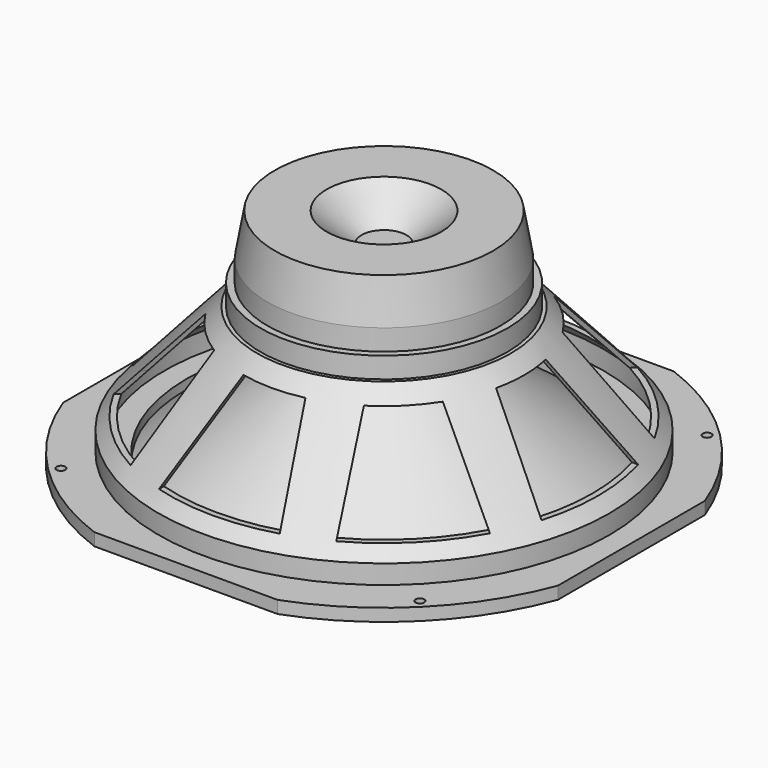
from build123d import *

# Parameters (mm, degrees)
F0_W            = 309.62
F0_H            = 309.62
F3_DEPTH        = 140.601
F5_D            = 5.5
F5_COPIES_COUNT = 4
F6_DEPTH        = 154.811
F6_COPIES_COUNT = 8


# Not quite as in the source:
# - a pattern or mirror of a feature is missing from the dataset's text; its kind, count and spacing are read off the source's solid


with BuildPart() as f2:
    # F1 (on Front) → F2 (revolve)
    with BuildSketch(Plane.XZ):
        with BuildLine():
            Line((68.279650833, 140.6), (35.8839115326, 140.6))
            Line((35.8839115326, 140.6), (14.0041140839, 122.5903257728))
            Line((14.0041140839, 122.5903257728), (0, 122.5903257728))
            Line((0, 122.5903257728), (0, 87.8334343433))
            Line((0, 87.8334343433), (24.2440421134, 87.8334343433))
            Line((24.2440421134, 87.8334343433), (75.8107602596, 87.8334343433))
            Line((75.8107602596, 87.8334343433), (137.3430937529, 19.6983087808))
            Line((137.3430937529, 19.6983087808), (137.3430937529, 7.8))
            Line((137.3430937529, 7.8), (123.4618676256, 7.8))
            Line((123.4618676256, 7.8), (123.4618676256, 2))
            ThreePointArc((123.4618676256, 2), (123.6694145774, 1.1128066334), (124.2489796953, 0.4097475457))
            ThreePointArc((124.2489796953, 0.4097475457), (126.3490609922, 0.2075469517), (127.4618676256, 2))
            ThreePointArc((127.4618676256, 2), (129.4618676256, 4), (131.4618676256, 2))
            ThreePointArc((131.4618676256, 2), (132.0476540633, 0.5857864376), (133.4618676256, 0))
            Line((133.4618676256, 0), (165.1, 0))
            Line((165.1, 0), (165.1, 7.8))
            Line((165.1, 7.8), (141, 7.8))
            Line((141, 7.8), (141, 19.6983087808))
            Line((141, 19.6983087808), (79.4676665068, 87.8334343433))
            Line((79.4676665068, 87.8334343433), (77.2199082971, 87.8334343433))
            Line((77.2199082971, 87.8334343433), (77.2199082971, 100.8985191584))
            Line((77.2199082971, 100.8985191584), (72.9740634561, 100.8985191584))
            Line((72.9740634561, 100.8985191584), (72.9740634561, 113.9636039734))
            Line((72.9740634561, 113.9636039734), (68.279650833, 140.6))
        make_face()
    revolve(axis=Axis((0, 0, 64.3603586431), (0, 0, 1)))

    # F0 (on Top) → F3 (intersect, through all)
    with BuildSketch(Plane.XY):
        Rectangle(F0_W, F0_H)
    extrude(amount=F3_DEPTH, mode=Mode.INTERSECT)

    # F5 (through all)
    with Locations(Plane(origin=(0, 0, 0), x_dir=(1, 0, 0), z_dir=(0, 0, -1))):
        with Locations((112.2532015134, -112.2532015134)):
            f5 = Hole(F5_D / 2)

    # F5_copies: F5 ×4 about axis
    f5_copies_axis = Axis((0, 0, 0), (0, 0, 1))
    for i in range(1, F5_COPIES_COUNT):
        add(f5.rotate(f5_copies_axis, i * 360 / F5_COPIES_COUNT), mode=Mode.SUBTRACT)

    # F1 (on Front) → F6 (cut, through all)
    with BuildSketch(Plane.XZ):
        with BuildLine():
            Line((19.4013845176, 78.6009654403), (0, 78.6009654403))
            Line((0, 78.6009654403), (0, 36.9858598114))
            ThreePointArc((0, 36.9858598114), (16.4033585457, 38.3463341411), (32.3584563521, 42.3905789372))
            Line((32.3584563521, 42.3905789372), (19.4013845176, 78.6009654403))
        make_face()
        Polygon((0, 36.9858598114), (0, 78.6009654403), (-19.4013845176, 78.6009654403), (-37.7621427178, 27.2892061621), (0, 27.2892061621), align=None)
        with BuildLine():
            ThreePointArc((32.3584563521, 42.3905789372), (16.4033585457, 38.3463341411), (0, 36.9858598114))
            Line((0, 36.9858598114), (0, 27.2892061621))
            Line((0, 27.2892061621), (37.7621427178, 27.2892061621))
            Line((37.7621427178, 27.2892061621), (32.3584563521, 42.3905789372))
        make_face()
    f6 = extrude(amount=-F6_DEPTH, mode=Mode.SUBTRACT)

    # F6_copies: F6 ×8 about axis
    f6_copies_axis = Axis((0, 0, 0), (0, 0, 1))
    for i in range(1, F6_COPIES_COUNT):
        add(f6.rotate(f6_copies_axis, i * 360 / F6_COPIES_COUNT), mode=Mode.SUBTRACT)


with BuildPart() as f7:
    # F1 (on Front) → F7 (revolve)
    with BuildSketch(Plane.XZ):
        with BuildLine():
            Line((24.2440421134, 87.8334343433), (0, 87.8334343433))
            Line((0, 87.8334343433), (0, 78.6009654403))
            Line((0, 78.6009654403), (19.4013845176, 78.6009654403))
            Line((19.4013845176, 78.6009654403), (32.3584563521, 42.3905789372))
            ThreePointArc((32.3584563521, 42.3905789372), (43.9102213021, 47.1911638175), (54.7688728633, 53.4023291611))
            Line((54.7688728633, 53.4023291611), (124.2489796953, 0.4097475457))
            ThreePointArc((124.2489796953, 0.4097475457), (123.6694145774, 1.1128066334), (123.4618676256, 2))
            Line((123.4618676256, 2), (24.2440421134, 77.6735842228))
            Line((24.2440421134, 77.6735842228), (24.2440421134, 87.8334343433))
        make_face()
        with BuildLine():
            Line((19.4013845176, 78.6009654403), (0, 78.6009654403))
            Line((0, 78.6009654403), (0, 36.9858598114))
            ThreePointArc((0, 36.9858598114), (16.4033585457, 38.3463341411), (32.3584563521, 42.3905789372))
            Line((32.3584563521, 42.3905789372), (19.4013845176, 78.6009654403))
        make_face()
    revolve(axis=Axis((0, 0, 64.3603586431), (0, 0, 1)))


solid = Compound([f2.part, f7.part])
